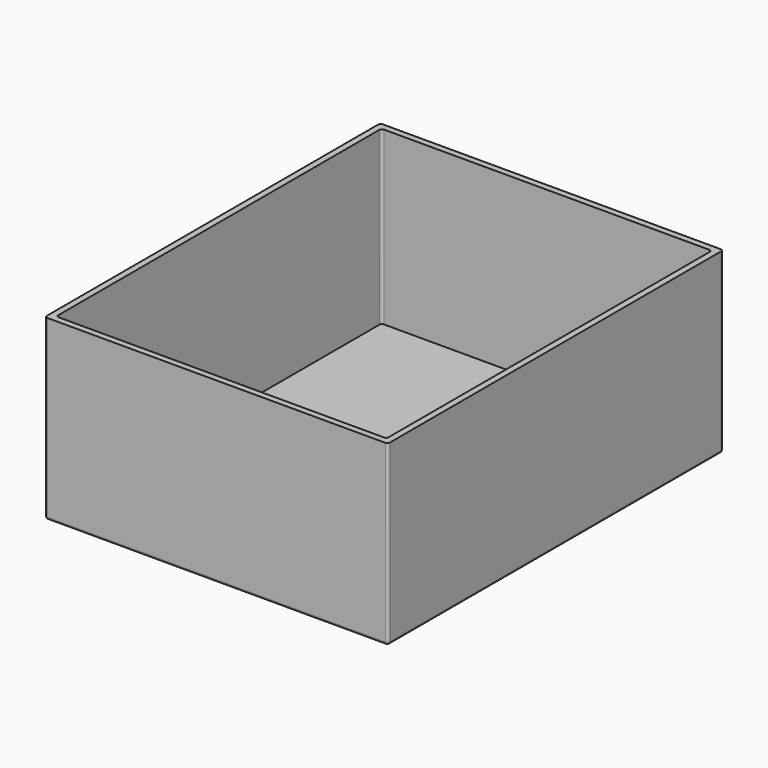
from build123d import *

# Parameters (mm, degrees)
F0_W     = 68.58
F0_H     = 83.82
F1_DEPTH = 35.56
F2_R     = 0.508
F3_T     = -1.27
F4_R     = 0.508


with BuildPart() as f1:
    # F0 (on Top) → F1 (new body)
    with BuildSketch(Plane.XY):
        with Locations((36.83, 44.45)):
            Rectangle(F0_W, F0_H)
    extrude(amount=F1_DEPTH)

    # F2
    f2_edges = [f1.edges().sort_by_distance(p)[0] for p in [
        (71.12, 2.54, 17.78),
        (71.12, 86.36, 17.78),
        (2.54, 2.54, 17.78),
        (2.54, 86.36, 17.78),
        (71.12, 44.45, 0),
        (2.54, 44.45, 0),
        (36.83, 2.54, 0),
        (36.83, 86.36, 0),
    ]]
    fillet(f2_edges, radius=F2_R)

    # F3
    f3_openings = [f1.faces().sort_by_distance(p)[0] for p in [
        (36.83, 44.45, 35.56),
    ]]
    offset(amount=F3_T, openings=f3_openings)

    # F4
    f4_edges = [f1.edges().sort_by_distance(p)[0] for p in [
        (3.81, 3.81, 18.415),
        (3.81, 85.09, 18.415),
        (69.85, 85.09, 18.415),
        (69.85, 3.81, 18.415),
    ]]
    fillet(f4_edges, radius=F4_R)


solid = f1.part
